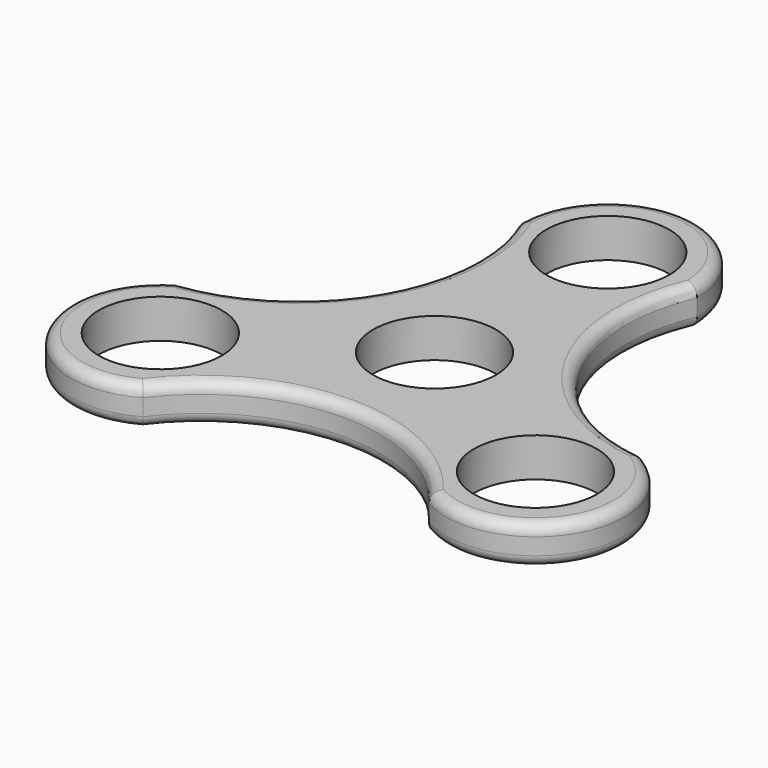
from build123d import *

# Parameters (mm, degrees)
F0_R         = 11.05
F1_DEPTH     = 7
F2_T2_ANGLE  = 215.755714617
F2_T4_ANGLE  = 215.755714617
F2_T6_ANGLE  = 215.755714617
F2_T8_ANGLE  = 215.755714617
F2_T10_ANGLE = 215.755714617
F2_T12_ANGLE = 215.755714617
F2_T14_ANGLE = 124.5631041465
F2_T16_ANGLE = 124.5631041465
F2_T18_ANGLE = 124.5631041465
F2_T20_ANGLE = 124.5631041465
F2_T22_ANGLE = 124.5631041465
F2_T24_ANGLE = 124.5631041465


# Not quite as in the source:
# - a fillet or chamfer that OpenCascade refuses, or shapes differently, is made with other operations: its cross-section is extruded or revolved along the edge and cut away or added
# - a feature names something its author has since deleted; it is built from what else it names


with BuildPart() as f1:
    # F0 (on Top) → F1 (new body)
    with BuildSketch(Plane.XY):
        with BuildLine():
            ThreePointArc((41.7566894774, -5.5752922693), (17.7217077983, 10.2316327678), (16.05, 38.95))
            ThreePointArc((16.05, 38.95), (0, 55), (-16.05, 38.95))
            ThreePointArc((-16.05, 38.95), (-17.7217077983, 10.2316327678), (-41.7566894774, -5.5752922693))
            ThreePointArc((-41.7566894774, -5.5752922693), (-47.6313972081, -27.5), (-25.7066894774, -33.3747077307))
            ThreePointArc((-25.7066894774, -33.3747077307), (0, -20.4632655356), (25.7066894774, -33.3747077307))
            ThreePointArc((25.7066894774, -33.3747077307), (47.6313972081, -27.5), (41.7566894774, -5.5752922693))
        make_face()
        with Locations((-33.7316894774, -19.475)):
            Circle(F0_R, mode=Mode.SUBTRACT)
        with Locations((33.7316894774, -19.475)):
            Circle(F0_R, mode=Mode.SUBTRACT)
        Circle(F0_R, mode=Mode.SUBTRACT)
        with Locations((0, 38.95)):
            Circle(F0_R, mode=Mode.SUBTRACT)
    extrude(amount=F1_DEPTH)

    # F2: fillet of radius 2 on 12 edges, made by hand

    # F2_s1 → F2_t2 (revolve, cut)
    with BuildSketch(Plane(origin=(11.3798385949, 35.279268365, 0), x_dir=(0, 0, 1), z_dir=(-0.306988839, -0.9517131147, 0))):
        with BuildLine():
            ThreePointArc((5, -4.0927847229), (6.4142135624, -3.5069982853), (7, -2.0927847229))
            Line((7, -2.0927847229), (7, -4.0927847229))
            Line((7, -4.0927847229), (5, -4.0927847229))
        make_face()
    revolve(axis=Axis((0, 38.95, 7), (0, 0, 1)), revolution_arc=F2_T2_ANGLE, mode=Mode.SUBTRACT)

    # F2_s3 → F2_t4 (revolve, cut)
    with BuildSketch(Plane(origin=(24.8628233335, -27.4948634967, 0), x_dir=(0, 0, 1), z_dir=(-0.670713315, 0.7417166906, 0))):
        with BuildLine():
            ThreePointArc((5, -4.0927847229), (6.4142135624, -3.5069982853), (7, -2.0927847229))
            Line((7, -2.0927847229), (7, -4.0927847229))
            Line((7, -4.0927847229), (5, -4.0927847229))
        make_face()
    revolve(axis=Axis((33.7316894774, -19.475, 7), (0, 0, 1)), revolution_arc=F2_T4_ANGLE, mode=Mode.SUBTRACT)

    # F2_s5 → F2_t6 (revolve, cut)
    with BuildSketch(Plane(origin=(-36.2426619285, -7.7844048683, 0), x_dir=(0, 0, 1), z_dir=(0.977702154, 0.2099964242, 0))):
        with BuildLine():
            ThreePointArc((5, -4.0927847229), (6.4142135624, -3.5069982853), (7, -2.0927847229))
            Line((7, -2.0927847229), (7, -4.0927847229))
            Line((7, -4.0927847229), (5, -4.0927847229))
        make_face()
    revolve(axis=Axis((-33.7316894774, -19.475, 7), (0, 0, 1)), revolution_arc=F2_T6_ANGLE, mode=Mode.SUBTRACT)

    # F2_s7 → F2_t8 (revolve, cut)
    with BuildSketch(Plane(origin=(-36.2426619285, -7.7844048683, 0), x_dir=(0, 0, 1), z_dir=(0.977702154, 0.2099964242, 0))):
        with BuildLine():
            ThreePointArc((2, -4.0927847229), (0.5857864376, -3.5069982853), (0, -2.0927847229))
            Line((0, -2.0927847229), (0, -4.0927847229))
            Line((0, -4.0927847229), (2, -4.0927847229))
        make_face()
    revolve(axis=Axis((-33.7316894774, -19.475, 0), (0, 0, 1)), revolution_arc=F2_T8_ANGLE, mode=Mode.SUBTRACT)

    # F2_s9 → F2_t10 (revolve, cut)
    with BuildSketch(Plane(origin=(11.3798385949, 35.279268365, 0), x_dir=(0, 0, 1), z_dir=(-0.306988839, -0.9517131147, 0))):
        with BuildLine():
            ThreePointArc((2, -4.0927847229), (0.5857864376, -3.5069982853), (0, -2.0927847229))
            Line((0, -2.0927847229), (0, -4.0927847229))
            Line((0, -4.0927847229), (2, -4.0927847229))
        make_face()
    revolve(axis=Axis((0, 38.95, 0), (0, 0, 1)), revolution_arc=F2_T10_ANGLE, mode=Mode.SUBTRACT)

    # F2_s11 → F2_t12 (revolve, cut)
    with BuildSketch(Plane(origin=(24.8628233335, -27.4948634967, 0), x_dir=(0, 0, 1), z_dir=(-0.670713315, 0.7417166906, 0))):
        with BuildLine():
            ThreePointArc((2, -4.0927847229), (0.5857864376, -3.5069982853), (0, -2.0927847229))
            Line((0, -2.0927847229), (0, -4.0927847229))
            Line((0, -4.0927847229), (2, -4.0927847229))
        make_face()
    revolve(axis=Axis((33.7316894774, -19.475, 0), (0, 0, 1)), revolution_arc=F2_T12_ANGLE, mode=Mode.SUBTRACT)

    # F2_s13 → F2_t14 (revolve, cut)
    with BuildSketch(Plane(origin=(-24.8262686526, 39.2992829747, 0), x_dir=(0, 0, 1), z_dir=(-0.5340801668, 0.8454338386, 0))):
        with BuildLine():
            ThreePointArc((2, 7.6229127052), (0.5857864376, 8.2086991428), (0, 9.6229127052))
            Line((0, 9.6229127052), (0, 7.6229127052))
            Line((0, 7.6229127052), (2, 7.6229127052))
        make_face()
    revolve(axis=Axis((-45.4749974503, 26.2550020193, 0), (0, 0, -1)), revolution_arc=F2_T14_ANGLE, mode=Mode.SUBTRACT)

    # F2_s15 → F2_t16 (revolve, cut)
    with BuildSketch(Plane(origin=(-24.8262686526, 39.2992829747, 0), x_dir=(0, 0, 1), z_dir=(-0.5340801668, 0.8454338386, 0))):
        with BuildLine():
            ThreePointArc((5, 7.6229127052), (6.4142135624, 8.2086991428), (7, 9.6229127052))
            Line((7, 9.6229127052), (7, 7.6229127052))
            Line((7, 7.6229127052), (5, 7.6229127052))
        make_face()
    revolve(axis=Axis((-45.4749974503, 26.2550020193, 7), (0, 0, -1)), revolution_arc=F2_T16_ANGLE, mode=Mode.SUBTRACT)

    # F2_s17 → F2_t18 (revolve, cut)
    with BuildSketch(Plane(origin=(46.4473117329, 1.850537847, 0), x_dir=(0, 0, 1), z_dir=(0.9992072648, 0.0398100728, 0))):
        with BuildLine():
            ThreePointArc((2, 7.6229127052), (0.5857864376, 8.2086991428), (0, 9.6229127052))
            Line((0, 9.6229127052), (0, 7.6229127052))
            Line((0, 7.6229127052), (2, 7.6229127052))
        make_face()
    revolve(axis=Axis((45.4749974503, 26.2550020193, 0), (0, 0, -1)), revolution_arc=F2_T18_ANGLE, mode=Mode.SUBTRACT)

    # F2_s19 → F2_t20 (revolve, cut)
    with BuildSketch(Plane(origin=(46.4473117329, 1.850537847, 0), x_dir=(0, 0, 1), z_dir=(0.9992072648, 0.0398100728, 0))):
        with BuildLine():
            ThreePointArc((5, 7.6229127052), (6.4142135624, 8.2086991428), (7, 9.6229127052))
            Line((7, 9.6229127052), (7, 7.6229127052))
            Line((7, 7.6229127052), (5, 7.6229127052))
        make_face()
    revolve(axis=Axis((45.4749974503, 26.2550020193, 7), (0, 0, -1)), revolution_arc=F2_T20_ANGLE, mode=Mode.SUBTRACT)

    # F2_s21 → F2_t22 (revolve, cut)
    with BuildSketch(Plane(origin=(-21.6210430802, -41.1498208217, 0), x_dir=(0, 0, 1), z_dir=(-0.4651270981, -0.8852439114, 0))):
        with BuildLine():
            ThreePointArc((5, 7.6229127052), (6.4142135624, 8.2086991428), (7, 9.6229127052))
            Line((7, 9.6229127052), (7, 7.6229127052))
            Line((7, 7.6229127052), (5, 7.6229127052))
        make_face()
    revolve(axis=Axis((0, -52.5100040386, 7), (0, 0, -1)), revolution_arc=F2_T22_ANGLE, mode=Mode.SUBTRACT)

    # F2_s23 → F2_t24 (revolve, cut)
    with BuildSketch(Plane(origin=(-21.6210430802, -41.1498208217, 0), x_dir=(0, 0, 1), z_dir=(-0.4651270981, -0.8852439114, 0))):
        with BuildLine():
            ThreePointArc((2, 7.6229127052), (0.5857864376, 8.2086991428), (0, 9.6229127052))
            Line((0, 9.6229127052), (0, 7.6229127052))
            Line((0, 7.6229127052), (2, 7.6229127052))
        make_face()
    revolve(axis=Axis((0, -52.5100040386, 0), (0, 0, -1)), revolution_arc=F2_T24_ANGLE, mode=Mode.SUBTRACT)


solid = f1.part
